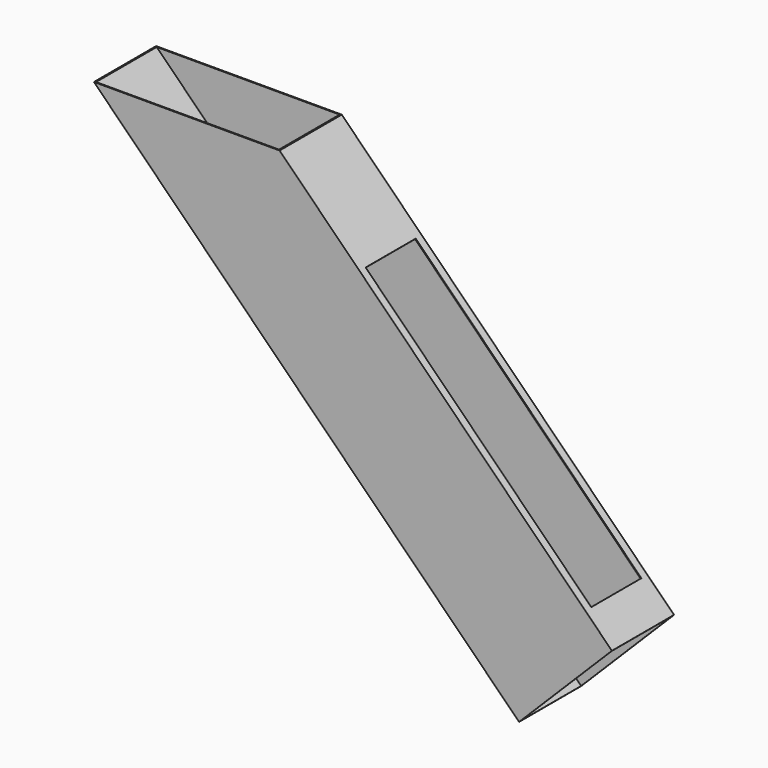
from build123d import *

# Parameters (mm, degrees)
F4_W      = 206
F4_H      = 348
F5_DEPTH  = 1800
F6_T      = -2.5
F7_W      = 1062.3749792576
F7_H      = 600.0114679337
F8_DEPTH  = 391.7381567773
F9_W      = 166
F9_H      = 846
F10_DEPTH = 12.5


with BuildPart() as f5:
    # F4 (on face) → F5 (new body)
    with BuildSketch(Plane(origin=(1004.0916292849, 0, -1004.0916292849), x_dir=(0, 1, 0), z_dir=(0.7071067812, 0, -0.7071067812))):
        Rectangle(F4_W, F4_H)
    extrude(amount=-F5_DEPTH)

    # F6
    f6_openings = [f5.faces().sort_by_distance(p)[0] for p in [
        (1004.091629, 0, -1004.091629),
    ]]
    offset(amount=F6_T, openings=f6_openings)

    # F7 (on Top) → F8 (cut, through all)
    with BuildSketch(Plane.XY):
        with Locations((39.5732372999, -20.192950964)):
            Rectangle(F7_W, F7_H)
    extrude(amount=F8_DEPTH, mode=Mode.SUBTRACT)

    # F9 (on face) → F10 (cut, symmetric)
    with BuildSketch(Plane(origin=(123.0365799265, 0, 123.0365799265), x_dir=(0, 1, 0), z_dir=(0.7071067812, 0, 0.7071067812))):
        with Locations((0, -897)):
            Rectangle(F9_W, F9_H)
    extrude(amount=F10_DEPTH, both=True, mode=Mode.SUBTRACT)


solid = f5.part
